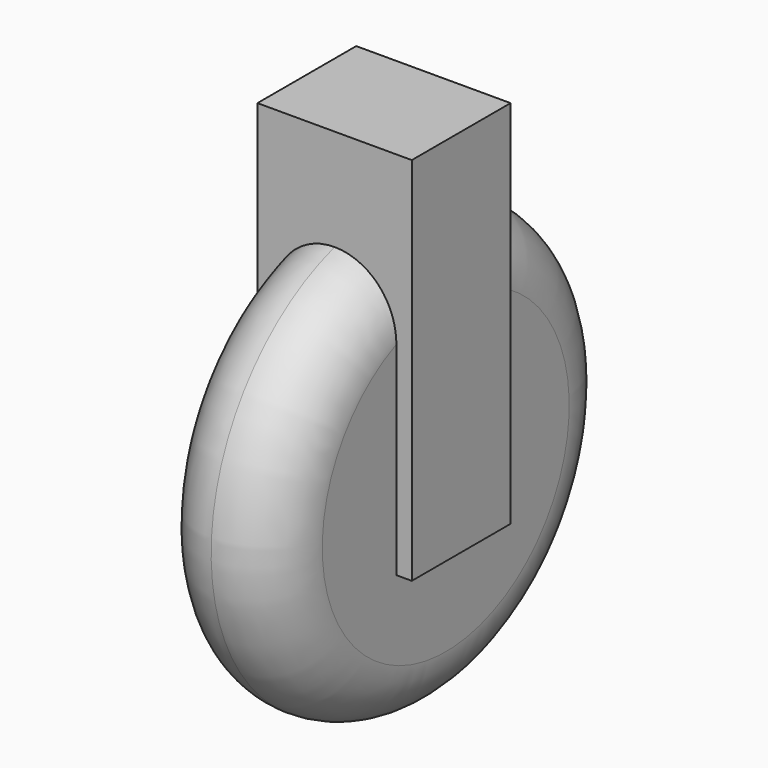
from build123d import *

# Parameters (mm, degrees)
F0_R     = 44.45
F0_R_2   = 6.35
F1_DEPTH = 12.7
F2_R     = 12.69999
F4_DEPTH = 12.7


# Not quite as in the source:
# - a fillet or chamfer is up to 0.001 mm smaller than in the source, because OpenCascade refuses the exact size


with BuildPart() as f1:
    # F0 (on Right) → F1 (new body, symmetric)
    with BuildSketch(Plane.YZ):
        Circle(F0_R)
        Circle(F0_R_2, mode=Mode.SUBTRACT)
    extrude(amount=F1_DEPTH, both=True)

    # F2 (radius 12.7 in the source; OpenCascade refuses exactly that, so slightly less here)
    f2_edges = [f1.edges().sort_by_distance(p)[0] for p in [
        (12.7, -44.45, 0),
        (-12.7, -44.45, 0),
    ]]
    fillet(f2_edges, radius=F2_R)

    # F3 (on Front) → F4 (join, symmetric)
    with BuildSketch(Plane.XZ):
        Polygon((15.875, 63.5), (-15.875, 63.5), (-15.875, 12.7), (-15.875, -12.7), (15.875, -12.7), (15.875, 12.7), align=None)
    extrude(amount=F4_DEPTH, both=True)


solid = f1.part
